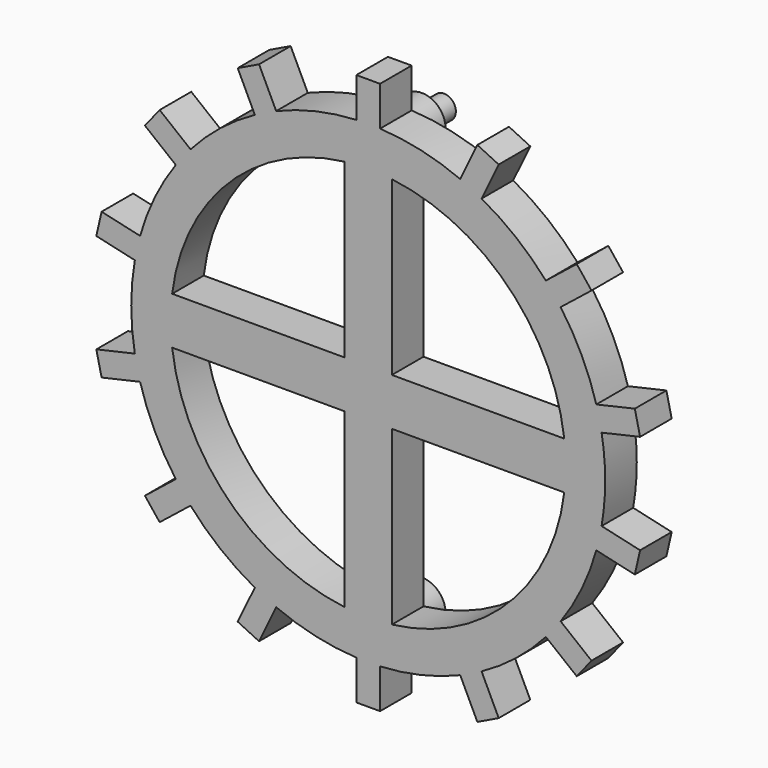
from build123d import *

# Parameters (mm, degrees)
F0_W     = 7.62
F0_H     = 7.62
F1_DEPTH = 3.175
F2_R     = 3.81
F3_DEPTH = 4.445
F4_R     = 1.905
F5_DEPTH = 4.445
F6_R     = 1.905
F7_DEPTH = 4.445


with BuildPart() as f1:
    # F0 (on Front) → F1 (new body, symmetric)
    with BuildSketch(Plane.XZ):
        with BuildLine():
            ThreePointArc((37.5221958358, -6.6102057198), (37.9552740824, -3.3177054311), (38.1, 0))
            ThreePointArc((38.1, 0), (37.9552740824, 3.3177054311), (37.5221958358, 6.6102057198))
            ThreePointArc((37.5221958358, 6.6102057198), (37.1447534541, 8.4780475837), (36.6743910775, 10.3246810652))
            ThreePointArc((36.6743910775, 10.3246810652), (34.3269138671, 16.5309704604), (30.9382695294, 22.2358601931))
            ThreePointArc((30.9382695294, 22.2358601931), (29.787779482, 23.7549614508), (28.5627733843, 25.2146381413))
            ThreePointArc((28.5627733843, 25.2146381413), (23.7549614508, 29.787779482), (18.2266395097, 33.4574298503))
            ThreePointArc((18.2266395097, 33.4574298503), (16.5309704604, 34.3269138671), (14.793948123, 35.1105268963))
            ThreePointArc((14.793948123, 35.1105268963), (8.4780475837, 37.1447534541), (1.905, 38.0523451971))
            ThreePointArc((1.905, 38.0523451971), (0, 38.1), (-1.905, 38.0523451971))
            ThreePointArc((-1.905, 38.0523451971), (-8.4780475837, 37.1447534541), (-14.793948123, 35.1105268963))
            ThreePointArc((-14.793948123, 35.1105268963), (-16.5309704604, 34.3269138671), (-18.2266395097, 33.4574298503))
            ThreePointArc((-18.2266395097, 33.4574298503), (-23.7549614508, 29.787779482), (-28.5627733843, 25.2146381413))
            ThreePointArc((-28.5627733843, 25.2146381413), (-29.787779482, 23.7549614508), (-30.9382695294, 22.2358601931))
            ThreePointArc((-30.9382695294, 22.2358601931), (-34.3269138671, 16.5309704604), (-36.6743910775, 10.3246810652))
            ThreePointArc((-36.6743910775, 10.3246810652), (-37.1447534541, 8.4780475837), (-37.5221958358, 6.6102057198))
            ThreePointArc((-37.5221958358, 6.6102057198), (-38.1, 0), (-37.5221958358, -6.6102057198))
            ThreePointArc((-37.5221958358, -6.6102057198), (-37.1447534541, -8.4780475837), (-36.6743910775, -10.3246810652))
            ThreePointArc((-36.6743910775, -10.3246810652), (-34.3269138671, -16.5309704604), (-30.9382695294, -22.2358601931))
            ThreePointArc((-30.9382695294, -22.2358601931), (-29.787779482, -23.7549614508), (-28.5627733843, -25.2146381413))
            ThreePointArc((-28.5627733843, -25.2146381413), (-23.7549614508, -29.787779482), (-18.2266395097, -33.4574298503))
            ThreePointArc((-18.2266395097, -33.4574298503), (-16.5309704604, -34.3269138671), (-14.793948123, -35.1105268963))
            ThreePointArc((-14.793948123, -35.1105268963), (-8.4780475837, -37.1447534541), (-1.905, -38.0523451971))
            ThreePointArc((-1.905, -38.0523451971), (0, -38.1), (1.905, -38.0523451971))
            ThreePointArc((1.905, -38.0523451971), (8.4780475837, -37.1447534541), (14.793948123, -35.1105268963))
            ThreePointArc((14.793948123, -35.1105268963), (16.5309704604, -34.3269138671), (18.2266395097, -33.4574298503))
            ThreePointArc((18.2266395097, -33.4574298503), (23.7549614508, -29.787779482), (28.5627733843, -25.2146381413))
            ThreePointArc((28.5627733843, -25.2146381413), (29.787779482, -23.7549614508), (30.9382695294, -22.2358601931))
            ThreePointArc((30.9382695294, -22.2358601931), (34.3269138671, -16.5309704604), (36.6743910775, -10.3246810652))
            ThreePointArc((36.6743910775, -10.3246810652), (37.1447534541, -8.4780475837), (37.5221958358, -6.6102057198))
        make_face()
        with BuildLine():
            ThreePointArc((31.5205710608, 3.81), (31.6925908627, 1.9084507878), (31.75, 0))
            ThreePointArc((31.75, 0), (31.6925908627, -1.9084507878), (31.5205710608, -3.81))
            ThreePointArc((31.5205710608, -3.81), (22.4506403027, -22.4506403027), (3.81, -31.5205710608))
            ThreePointArc((3.81, -31.5205710608), (0, -31.75), (-3.81, -31.5205710608))
            ThreePointArc((-3.81, -31.5205710608), (-22.4506403027, -22.4506403027), (-31.5205710608, -3.81))
            ThreePointArc((-31.5205710608, -3.81), (-31.75, 0), (-31.5205710608, 3.81))
            ThreePointArc((-31.5205710608, 3.81), (-22.4506403027, 22.4506403027), (-3.81, 31.5205710608))
            ThreePointArc((-3.81, 31.5205710608), (0, 31.75), (3.81, 31.5205710608))
            ThreePointArc((3.81, 31.5205710608), (22.4506403027, 22.4506403027), (31.5205710608, 3.81))
        make_face(mode=Mode.SUBTRACT)
        with BuildLine():
            ThreePointArc((36.6743910775, 10.3246810652), (37.1447534541, 8.4780475837), (37.5221958358, 6.6102057198))
            Line((37.5221958358, 6.6102057198), (43.7129880782, 8.0232136504))
            Line((43.7129880782, 8.0232136504), (42.8651833198, 11.7376889958))
            Line((42.8651833198, 11.7376889958), (36.6743910775, 10.3246810652))
        make_face()
        with BuildLine():
            Line((43.7129880782, -8.0232136504), (37.5221958358, -6.6102057198))
            ThreePointArc((37.5221958358, -6.6102057198), (37.1447534541, -8.4780475837), (36.6743910775, -10.3246810652))
            Line((36.6743910775, -10.3246810652), (42.8651833198, -11.7376889958))
            Line((42.8651833198, -11.7376889958), (43.7129880782, -8.0232136504))
        make_face()
        with BuildLine():
            ThreePointArc((28.5627733843, 25.2146381413), (29.787779482, 23.7549614508), (30.9382695294, 22.2358601931))
            Line((30.9382695294, 22.2358601931), (35.9028994431, 26.1950204349))
            Line((35.9028994431, 26.1950204349), (33.527403298, 29.1737983831))
            Line((33.527403298, 29.1737983831), (28.5627733843, 25.2146381413))
        make_face()
        with BuildLine():
            Line((35.9028994431, -26.1950204349), (30.9382695294, -22.2358601931))
            ThreePointArc((30.9382695294, -22.2358601931), (29.787779482, -23.7549614508), (28.5627733843, -25.2146381413))
            Line((28.5627733843, -25.2146381413), (33.527403298, -29.1737983831))
            Line((33.527403298, -29.1737983831), (35.9028994431, -26.1950204349))
        make_face()
        with BuildLine():
            ThreePointArc((14.793948123, 35.1105268963), (16.5309704604, 34.3269138671), (18.2266395097, 33.4574298503))
            Line((18.2266395097, 33.4574298503), (20.9818012531, 39.1785821614))
            Line((20.9818012531, 39.1785821614), (17.5491098664, 40.8316792075))
            Line((17.5491098664, 40.8316792075), (14.793948123, 35.1105268963))
        make_face()
        with BuildLine():
            Line((20.9818012531, -39.1785821614), (18.2266395097, -33.4574298503))
            ThreePointArc((18.2266395097, -33.4574298503), (16.5309704604, -34.3269138671), (14.793948123, -35.1105268963))
            Line((14.793948123, -35.1105268963), (17.5491098664, -40.8316792075))
            Line((17.5491098664, -40.8316792075), (20.9818012531, -39.1785821614))
        make_face()
        with BuildLine():
            ThreePointArc((-1.905, 38.0523451971), (0, 38.1), (1.905, 38.0523451971))
            Line((1.905, 38.0523451971), (1.905, 44.4023451971))
            Line((1.905, 44.4023451971), (-1.905, 44.4023451971))
            Line((-1.905, 44.4023451971), (-1.905, 38.0523451971))
        make_face()
        with BuildLine():
            Line((1.905, -44.4023451971), (1.905, -38.0523451971))
            ThreePointArc((1.905, -38.0523451971), (0, -38.1), (-1.905, -38.0523451971))
            Line((-1.905, -38.0523451971), (-1.905, -44.4023451971))
            Line((-1.905, -44.4023451971), (1.905, -44.4023451971))
        make_face()
        with BuildLine():
            ThreePointArc((-18.2266395097, 33.4574298503), (-16.5309704604, 34.3269138671), (-14.793948123, 35.1105268963))
            Line((-14.793948123, 35.1105268963), (-17.5491098664, 40.8316792075))
            Line((-17.5491098664, 40.8316792075), (-20.9818012531, 39.1785821614))
            Line((-20.9818012531, 39.1785821614), (-18.2266395097, 33.4574298503))
        make_face()
        with BuildLine():
            Line((-17.5491098664, -40.8316792075), (-14.793948123, -35.1105268963))
            ThreePointArc((-14.793948123, -35.1105268963), (-16.5309704604, -34.3269138671), (-18.2266395097, -33.4574298503))
            Line((-18.2266395097, -33.4574298503), (-20.9818012531, -39.1785821614))
            Line((-20.9818012531, -39.1785821614), (-17.5491098664, -40.8316792075))
        make_face()
        with BuildLine():
            ThreePointArc((-30.9382695294, 22.2358601931), (-29.787779482, 23.7549614508), (-28.5627733843, 25.2146381413))
            Line((-28.5627733843, 25.2146381413), (-33.527403298, 29.1737983831))
            Line((-33.527403298, 29.1737983831), (-35.9028994431, 26.1950204349))
            Line((-35.9028994431, 26.1950204349), (-30.9382695294, 22.2358601931))
        make_face()
        with BuildLine():
            Line((-33.527403298, -29.1737983831), (-28.5627733843, -25.2146381413))
            ThreePointArc((-28.5627733843, -25.2146381413), (-29.787779482, -23.7549614508), (-30.9382695294, -22.2358601931))
            Line((-30.9382695294, -22.2358601931), (-35.9028994431, -26.1950204349))
            Line((-35.9028994431, -26.1950204349), (-33.527403298, -29.1737983831))
        make_face()
        with BuildLine():
            ThreePointArc((-37.5221958358, 6.6102057198), (-37.1447534541, 8.4780475837), (-36.6743910775, 10.3246810652))
            Line((-36.6743910775, 10.3246810652), (-42.8651833198, 11.7376889958))
            Line((-42.8651833198, 11.7376889958), (-43.7129880782, 8.0232136504))
            Line((-43.7129880782, 8.0232136504), (-37.5221958358, 6.6102057198))
        make_face()
        with BuildLine():
            Line((-42.8651833198, -11.7376889958), (-36.6743910775, -10.3246810652))
            ThreePointArc((-36.6743910775, -10.3246810652), (-37.1447534541, -8.4780475837), (-37.5221958358, -6.6102057198))
            Line((-37.5221958358, -6.6102057198), (-43.7129880782, -8.0232136504))
            Line((-43.7129880782, -8.0232136504), (-42.8651833198, -11.7376889958))
        make_face()
        with BuildLine():
            ThreePointArc((31.5205710608, -3.81), (31.6925908627, -1.9084507878), (31.75, 0))
            ThreePointArc((31.75, 0), (31.6925908627, 1.9084507878), (31.5205710608, 3.81))
            Line((31.5205710608, 3.81), (3.81, 3.81))
            Line((3.81, 3.81), (3.81, -3.81))
            Line((3.81, -3.81), (31.5205710608, -3.81))
        make_face()
        with BuildLine():
            Line((3.81, 3.81), (3.81, 31.5205710608))
            ThreePointArc((3.81, 31.5205710608), (0, 31.75), (-3.81, 31.5205710608))
            Line((-3.81, 31.5205710608), (-3.81, 3.81))
            Line((-3.81, 3.81), (3.81, 3.81))
        make_face()
        Rectangle(F0_W, F0_H)
        with BuildLine():
            ThreePointArc((-3.81, -31.5205710608), (0, -31.75), (3.81, -31.5205710608))
            Line((3.81, -31.5205710608), (3.81, -3.81))
            Line((3.81, -3.81), (-3.81, -3.81))
            Line((-3.81, -3.81), (-3.81, -31.5205710608))
        make_face()
        with BuildLine():
            Line((-3.81, -3.81), (-3.81, 3.81))
            Line((-3.81, 3.81), (-31.5205710608, 3.81))
            ThreePointArc((-31.5205710608, 3.81), (-31.75, 0), (-31.5205710608, -3.81))
            Line((-31.5205710608, -3.81), (-3.81, -3.81))
        make_face()
    extrude(amount=F1_DEPTH, both=True)

    # F2 (on face) → F3 (join)
    with BuildSketch(Plane(origin=(0, 3.175, 0), x_dir=(-1, 0, 0), z_dir=(0, 1, 0))):
        with Locations((0, 34.29)):
            Circle(F2_R)
        with Locations((0, -34.29)):
            Circle(F2_R)
    extrude(amount=F3_DEPTH)

    # F4 (on face) → F5 (join)
    with BuildSketch(Plane(origin=(0, 7.62, 0), x_dir=(-1, 0, 0), z_dir=(0, 1, 0))):
        with Locations((0, 34.29)):
            Circle(F4_R)
    extrude(amount=F5_DEPTH)

    # F6 (on face) → F7 (cut)
    with BuildSketch(Plane(origin=(0, 7.62, 0), x_dir=(-1, 0, 0), z_dir=(0, 1, 0))):
        with Locations((0, -34.29)):
            Circle(F6_R)
    extrude(amount=-F7_DEPTH, mode=Mode.SUBTRACT)


solid = f1.part
